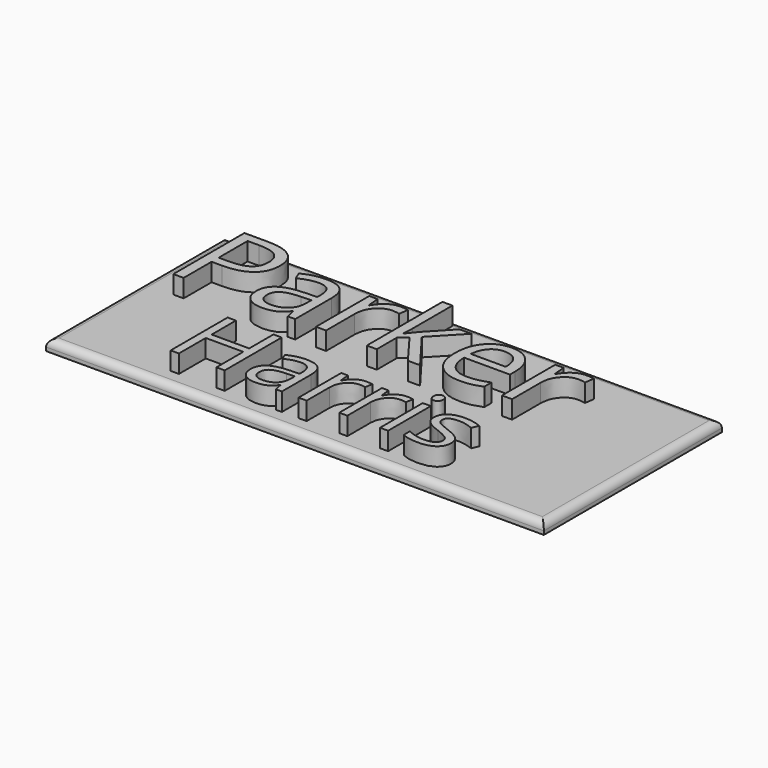
from build123d import *

# Parameters (mm, degrees)
F1_TEXT_SIZE = 27.6443962422
F0_TEXT_SIZE = 34.4870686402
F2_DEPTH     = 8
F3_W         = 137.9094868898
F3_H         = 61.6810359061
F4_DEPTH     = 3
F5_R         = 2


# Not quite as in the source:
# - Text() gives the source's letters only with a copy of the font that has no kerning and outlines rounded to 1/6400 em; it was checked with that copy


with BuildPart() as f2:
    # F1 (on Top) + F0 (on Top) → F2 (new body)
    with BuildSketch(Plane.XY):
        with Locations((-42.6831151708, -27.2995224223)):
            Text('Harris', F1_TEXT_SIZE, font='Open Sans', text_align=(TextAlign.LEFT, TextAlign.BOTTOM))
    with BuildSketch(Plane.XY):
        with Locations((-65.2419244871, 0.9872718947)):
            Text('Parker', F0_TEXT_SIZE, font='Open Sans', text_align=(TextAlign.LEFT, TextAlign.BOTTOM))
    extrude(amount=F2_DEPTH)


with BuildPart() as f4:
    # F3 (on Top) → F4 (new body)
    with BuildSketch(Plane.XY):
        with Locations((-1.4547407627, -1.5517231077)):
            Rectangle(F3_W, F3_H)
    extrude(amount=F4_DEPTH)

    # F5
    f5_edges = [f4.edges().sort_by_distance(p)[0] for p in [
        (-1.454741, -32.392241, 3),
        (67.500003, -1.551723, 3),
        (-1.454741, 29.288795, 3),
        (-70.409484, -1.551723, 3),
    ]]
    fillet(f5_edges, radius=F5_R)


solid = Compound([f2.part, f4.part])
